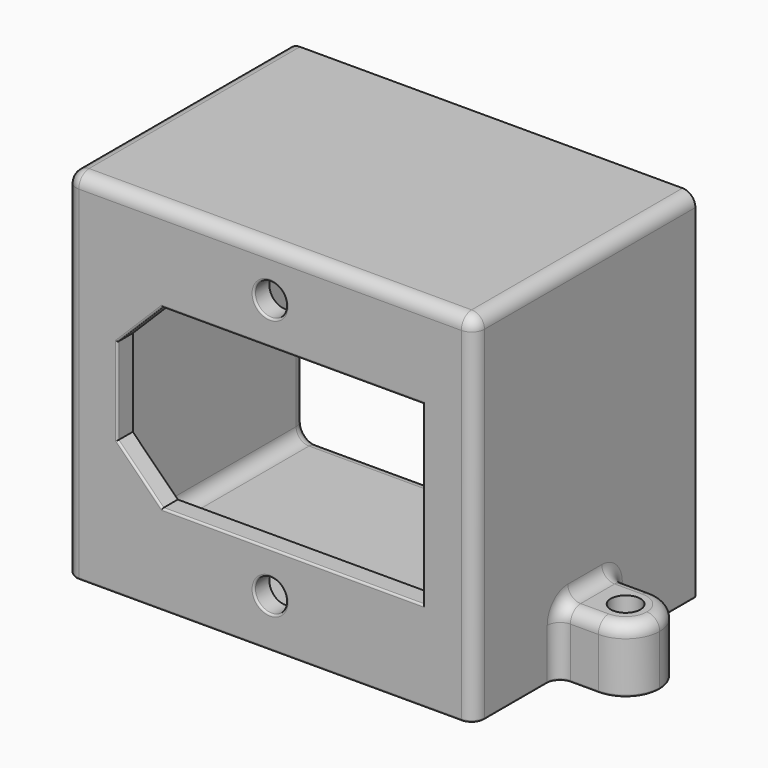
from build123d import *

# Parameters (mm, degrees)
F0_W     = 63.5
F0_H     = 55.5
F0_W_2   = 57.5
F0_H_2   = 50.2559055118
F0_R     = 2.5
F0_W_3   = 47.5
F0_H_3   = 27.5
F1_DEPTH = 3
F2_SIZE  = 7
F3_DEPTH = 40
F4_R     = 2.3
F5_DEPTH = 10
F6_R     = 2
F7_R     = 0.3


with BuildPart() as f1:
    # F0 (on Front) → F1 (new body)
    with BuildSketch(Plane.XZ):
        with Locations((-31.75, 27.75)):
            Rectangle(F0_W, F0_H)
        with Locations((-31.75, 27.75)):
            Rectangle(F0_W_2, F0_H_2, mode=Mode.SUBTRACT)
        with Locations((-31.75, 27.75)):
            Rectangle(F0_W_2, F0_H_2)
        with Locations((-31.75, 7.5)):
            Circle(F0_R, mode=Mode.SUBTRACT)
        with Locations((-31.75, 27.75)):
            Rectangle(F0_W_3, F0_H_3, mode=Mode.SUBTRACT)
        with Locations((-31.75, 48)):
            Circle(F0_R, mode=Mode.SUBTRACT)
    extrude(amount=F1_DEPTH)

    # F2
    f2_edges = [f1.edges().sort_by_distance(p)[0] for p in [
        (-55.5, -1.5, 41.5),
        (-55.5, -1.5, 14),
    ]]
    chamfer(f2_edges, length=F2_SIZE)

    # F0 (on Front) → F3 (join)
    with BuildSketch(Plane.XZ):
        with Locations((-31.75, 27.75)):
            Rectangle(F0_W, F0_H)
        with Locations((-31.75, 27.75)):
            Rectangle(F0_W_2, F0_H_2, mode=Mode.SUBTRACT)
    extrude(amount=-F3_DEPTH)

    # F4 (on face) → F5 (join)
    with BuildSketch(Plane(origin=(0, 0, 0), x_dir=(1, 0, 0), z_dir=(0, 0, -1))):
        with BuildLine():
            ThreePointArc((-69.85, -23.8), (-66.1023340597, -22.2476659403), (-64.55, -18.5))
            ThreePointArc((-64.55, -18.5), (-66.1023340597, -14.7523340597), (-69.85, -13.2))
            ThreePointArc((-69.85, -13.2), (-75.15, -18.5), (-69.85, -23.8))
        make_face()
        with Locations((-69.85, -18.5)):
            Circle(F4_R, mode=Mode.SUBTRACT)
        with BuildLine():
            ThreePointArc((6.35, -23.8), (10.0976659403, -22.2476659403), (11.65, -18.5))
            ThreePointArc((11.65, -18.5), (10.0976659403, -14.7523340597), (6.35, -13.2))
            ThreePointArc((6.35, -13.2), (1.05, -18.5), (6.35, -23.8))
        make_face()
        with Locations((6.35, -18.5)):
            Circle(F4_R, mode=Mode.SUBTRACT)
        with BuildLine():
            ThreePointArc((-69.85, -13.2), (-66.1023340597, -14.7523340597), (-64.55, -18.5))
            ThreePointArc((-64.55, -18.5), (-66.1023340597, -22.2476659403), (-69.85, -23.8))
            Line((-69.85, -23.8), (-63.5, -23.8))
            Line((-63.5, -23.8), (-63.5, -13.2))
            Line((-63.5, -13.2), (-69.85, -13.2))
        make_face()
        with BuildLine():
            Line((6.35, -13.2), (0, -13.2))
            Line((0, -13.2), (0, -23.8))
            Line((0, -23.8), (6.35, -23.8))
            ThreePointArc((6.35, -23.8), (1.05, -18.5), (6.35, -13.2))
        make_face()
    extrude(amount=-F5_DEPTH)

    # F6
    f6_edges = [f1.edges().sort_by_distance(p)[0] for p in [
        (-3, 20, 52.877953),
        (-3, 20, 2.622047),
        (-3, 0, 27.75),
        (-3, 40, 27.75),
        (-60.5, 20, 2.622047),
        (-31.75, 0, 2.622047),
        (-31.75, 40, 2.622047),
        (-60.5, 20, 52.877953),
        (-31.75, 0, 52.877953),
        (-31.75, 40, 52.877953),
        (-60.5, 0, 27.75),
        (-60.5, 40, 27.75),
        (-63.5, 18.5, 55.5),
        (-75.15, 18.5, 10),
        (-31.75, -3, 55.5),
        (0, 18.5, 55.5),
        (11.65, 18.5, 10),
        (0, -3, 27.75),
        (-63.5, -3, 27.75),
        (0, 13.2, 5),
        (0, 18.5, 10),
        (0, 23.8, 5),
        (-63.5, 23.8, 5),
        (-63.5, 18.5, 10),
        (-63.5, 13.2, 5),
        (3.175, 13.2, 10),
        (3.175, 23.8, 10),
        (-66.675, 23.8, 10),
        (-66.675, 13.2, 10),
    ]]
    fillet(f6_edges, radius=F6_R)

    # F7
    f7_edges = [f1.edges().sort_by_distance(p)[0] for p in [
        (-31.75, -3, 0),
        (-61.5, -3, 26.75),
        (-2, -3, 26.75),
        (-31.75, -3, 53.5),
        (-28.25, -3, 14),
        (-52, -3, 17.5),
        (-8, -3, 27.75),
        (-55.5, -3, 27.75),
        (-28.25, -3, 41.5),
        (-52, -3, 38),
        (-34.25, -3, 48),
        (-34.25, -3, 7.5),
        (-63.5, 5.1, 0),
        (-62.914214, -2.414214, 0),
        (-64.085786, 12.614214, 0),
        (-67.675, 13.2, 0),
        (-0.585786, -2.414214, 0),
        (-75.15, 18.5, 0),
        (0, 5.1, 0),
        (-67.675, 23.8, 0),
        (0.585786, 12.614214, 0),
        (-64.085786, 24.385786, 0),
        (4.175, 13.2, 0),
        (-63.5, 32.9, 0),
        (11.65, 18.5, 0),
        (4.175, 23.8, 0),
        (0, 32.9, 0),
        (0.585786, 24.385786, 0),
    ]]
    fillet(f7_edges, radius=F7_R)


solid = f1.part
